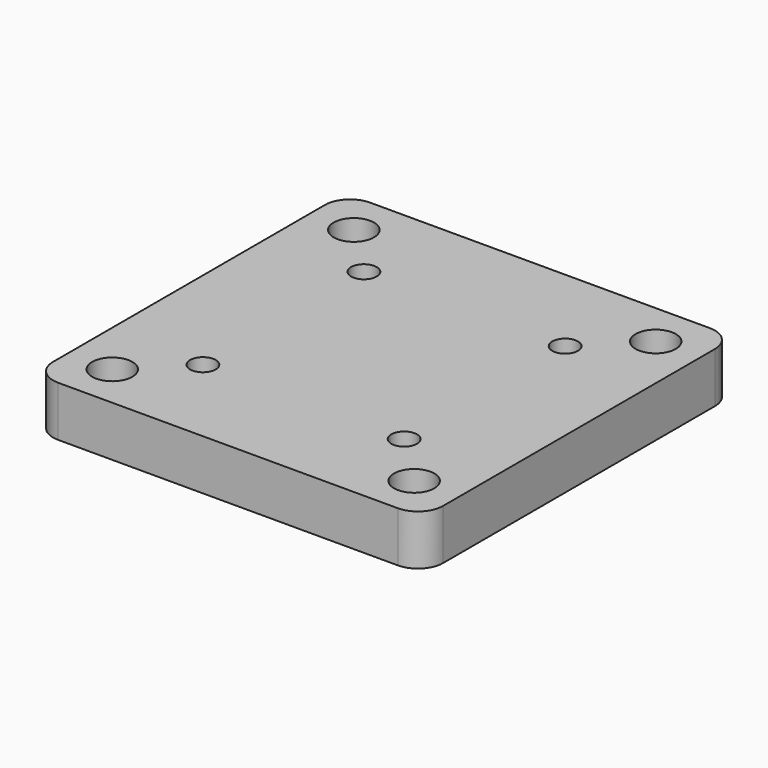
from build123d import *

# Parameters (mm, degrees)
F0_W     = 77.51
F0_H     = 77.519
F0_R     = 4
F0_R_2   = 5
F0_R_3   = 2.55
F1_DEPTH = 10
F2_R     = 5
F3_DEPTH = 4


# Not quite as in the source:
# - a feature names something its author has since deleted; it is built from what else it names


with BuildPart() as f1:
    # F0 (on Top) → F1 (new body)
    with BuildSketch(Plane.XY):
        Rectangle(F0_W, F0_H)
        with Locations((-30, -29.9995)):
            Circle(F0_R, mode=Mode.SUBTRACT)
        with Locations((-20, -19.9995)):
            Circle(F0_R_2, mode=Mode.SUBTRACT)
        with Locations((30, -29.9995)):
            Circle(F0_R, mode=Mode.SUBTRACT)
        with Locations((20, -19.9995)):
            Circle(F0_R_2, mode=Mode.SUBTRACT)
        with Locations((-20, 19.9995)):
            Circle(F0_R_2, mode=Mode.SUBTRACT)
        with Locations((-30, 29.9995)):
            Circle(F0_R, mode=Mode.SUBTRACT)
        with Locations((20, 19.9995)):
            Circle(F0_R_2, mode=Mode.SUBTRACT)
        with Locations((30, 29.9995)):
            Circle(F0_R, mode=Mode.SUBTRACT)
        with Locations((-20, 19.9995)):
            Circle(F0_R_2)
        with Locations((-20, 19.9995)):
            Circle(F0_R_3, mode=Mode.SUBTRACT)
        with Locations((20, 19.9995)):
            Circle(F0_R_2)
        with Locations((20, 19.9995)):
            Circle(F0_R_3, mode=Mode.SUBTRACT)
        with Locations((20, -19.9995)):
            Circle(F0_R_2)
        with Locations((20, -19.9995)):
            Circle(F0_R_3, mode=Mode.SUBTRACT)
        with Locations((-20, -19.9995)):
            Circle(F0_R_2)
        with Locations((-20, -19.9995)):
            Circle(F0_R_3, mode=Mode.SUBTRACT)
    extrude(amount=F1_DEPTH)

    # F2
    f2_edges = [f1.edges().sort_by_distance(p)[0] for p in [
        (38.755, -38.7595, 5),
        (-38.755, -38.7595, 5),
        (38.755, 38.7595, 5),
        (-38.755, 38.7595, 5),
    ]]
    fillet(f2_edges, radius=F2_R)

    # F0 (on Top) → F3 (cut)
    with BuildSketch(Plane.XY):
        with Locations((-20, 19.9995)):
            Circle(F0_R_2)
        with Locations((-20, 19.9995)):
            Circle(F0_R_3, mode=Mode.SUBTRACT)
        with Locations((20, 19.9995)):
            Circle(F0_R_2)
        with Locations((20, 19.9995)):
            Circle(F0_R_3, mode=Mode.SUBTRACT)
        with Locations((-20, -19.9995)):
            Circle(F0_R_2)
        with Locations((-20, -19.9995)):
            Circle(F0_R_3, mode=Mode.SUBTRACT)
        with Locations((20, -19.9995)):
            Circle(F0_R_2)
        with Locations((20, -19.9995)):
            Circle(F0_R_3, mode=Mode.SUBTRACT)
    extrude(amount=F3_DEPTH, mode=Mode.SUBTRACT)


solid = f1.part
